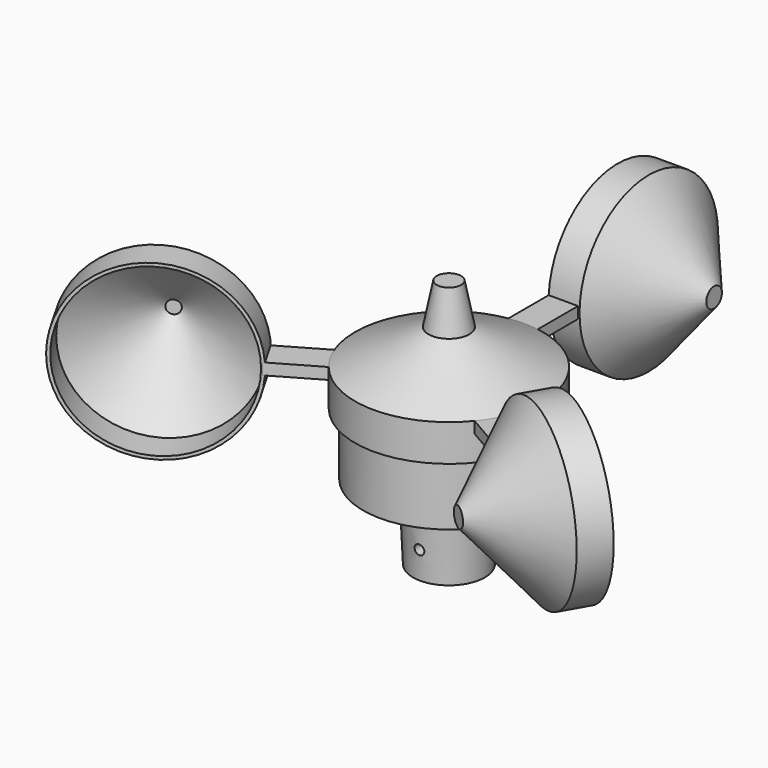
from build123d import *

# Parameters (mm, degrees)
F0_R       = 11
F2_R       = 12
F4_R       = 6.35
F5_R       = 6.35
F7_R       = 26.25
F8_DEPTH   = 19
F9_R       = 28.75
F10_DEPTH  = 9.5
F13_DEPTH  = 1.75
F15_R      = 28.75
F17_DEPTH  = 1.75
F17_FACE_R = 28.75
F16_R      = 6.25
F19_R      = 6.25
F21_R      = 3.75
F23_R      = 26.5
F23_R_2    = 25.5
F24_DEPTH  = 9.5
F27_R      = 26.5
F26_R      = 3
F30_R      = 2
F31_R      = 25.5
F34_COUNT  = 3
F35_R      = 1.5
F36_DEPTH  = 12.5
F37_R      = 6.35
F38_DEPTH  = 9.5


with BuildPart() as f3:
    # F0 (on Top) → F3 section 0
    with BuildSketch(Plane.XY):
        Circle(F0_R)
    # F2 (on offset) → F3 section 1
    with BuildSketch(Plane.XY.offset(23)):
        Circle(F2_R)
    loft()

    # F4 (on face) → F6 section 0
    with BuildSketch(Plane(origin=(0, 0, 0), x_dir=(1, 0, 0), z_dir=(0, 0, -1))):
        Circle(F4_R)
    # F5 (on face) → F6 section 1
    with BuildSketch(Plane.XY.offset(23)):
        Circle(F5_R)
    loft(mode=Mode.SUBTRACT)

    # F7 (on face) → F8 (join)
    with BuildSketch(Plane.XY.offset(23)):
        Circle(F7_R)
    extrude(amount=F8_DEPTH)

    # F9 (on face) → F10 (join)
    with BuildSketch(Plane.XY.offset(42)):
        Circle(F9_R)
    extrude(amount=F10_DEPTH)

    # F12 (on face) → F13 (join, symmetric)
    with BuildSketch(Plane.XY.offset(51.5)):
        Polygon((-4.5, 44.75), (-4.5, 28.3956422713), (-4.5, 22), (4.5, 22), (4.5, 28.3956422713), (4.5, 44.75), (0, 44.75), align=None)
        Polygon((-21.3025588833, -7.102885683), (-26.8413475637, -10.3007068186), (-40.6977540243, -18.3007068186), (-36.1977540243, -26.0949354527), (-22.3413475637, -18.0949354527), (-16.8025588833, -14.897114317), align=None)
        Polygon((16.8025588833, -14.897114317), (22.3413475637, -18.0949354527), (36.1977540243, -26.0949354527), (40.6977540243, -18.3007068186), (26.8413475637, -10.3007068186), (21.3025588833, -7.102885683), align=None)
    extrude(amount=F13_DEPTH, both=True)



with BuildPart() as f17:
    # F15 (on face) → F17 (new body)
    with BuildSketch(Plane.XY.offset(51.5)):
        Circle(F15_R)
    extrude(amount=F17_DEPTH)


with BuildPart() as f18:
    # F17_face (on face) → F18 section 0
    with BuildSketch(Plane.XY.offset(53.25)):
        Circle(F17_FACE_R)
    # F16 (on offset) → F18 section 1
    with BuildSketch(Plane.XY.offset(64)):
        Circle(F16_R)
    loft()


with BuildPart() as f3_1:
    add(f3.part)

    add(f17.part)  # F22 merges F17

    add(f18.part)  # F22 merges F18
    # F19 (on face) → F22 section 0
    with BuildSketch(Plane.XY.offset(64)):
        Circle(F19_R)
    # F21 (on offset) → F22 section 1
    with BuildSketch(Plane.XY.offset(76.5)):
        Circle(F21_R)
    loft()



with BuildPart() as f24:
    # F23 (on face) → F24 (new body)
    with BuildSketch(Plane(origin=(-4.5, 0, 0), x_dir=(0, -1, 0), z_dir=(-1, 0, 0))):
        with Locations((-70.25, 51.5)):
            Circle(F23_R)
        with Locations((-70.25, 51.5)):
            Circle(F23_R_2, mode=Mode.SUBTRACT)
    extrude(amount=-F24_DEPTH)


with BuildPart() as f3_2:
    add(f3_1.part)

    add(f24.part)  # F28 merges F24
    # F27 (on face) → F28 section 0
    with BuildSketch(Plane.YZ.offset(5)):
        with Locations((70.25, 51.5)):
            Circle(F27_R)
    # F26 (on offset) → F28 section 1
    with BuildSketch(Plane.YZ.offset(25)):
        with Locations((70.25, 51.5)):
            Circle(F26_R)
    loft()

    # F30 (on offset) → F32 section 0
    with BuildSketch(Plane.YZ.offset(24)):
        with Locations((70.25, 51.5)):
            Circle(F30_R)
    # F31 (on face) → F32 section 1
    with BuildSketch(Plane(origin=(5, 0, 0), x_dir=(0, -1, 0), z_dir=(-1, 0, 0))):
        with Locations((-70.25, 51.5)):
            Circle(F31_R)
    loft(mode=Mode.SUBTRACT)


with BuildPart() as f34_1:
    # F34: instance of F3
    add(f3_2.part.rotate(Axis((0, 0, 40.5513271689), (0, 0, 1)), 1 * 360 / F34_COUNT))


with BuildPart() as f34_2:
    # F34: instance of F3
    add(f3_2.part.rotate(Axis((0, 0, 40.5513271689), (0, 0, 1)), 2 * 360 / F34_COUNT))


with BuildPart() as f36_tool:
    # F35 (on Front) → F36 (new body, symmetric)
    with BuildSketch(Plane.XZ):
        with Locations((0, 8.5)):
            Circle(F35_R)
    extrude(amount=F36_DEPTH, both=True)


with BuildPart() as f3_3:
    add(f3_2.part)

    # F36: cut by f36_tool
    add(f36_tool.part, mode=Mode.SUBTRACT)



with BuildPart() as f34_1_1:
    add(f34_1.part)

    # F36: cut by f36_tool
    add(f36_tool.part, mode=Mode.SUBTRACT)


with BuildPart() as f34_2_1:
    add(f34_2.part)

    # F36: cut by f36_tool
    add(f36_tool.part, mode=Mode.SUBTRACT)


with BuildPart() as f3_4:
    add(f3_3.part)

    add(f34_1_1.part)  # F38 merges F34_1

    add(f34_2_1.part)  # F38 merges F34_2
    # F37 (on face) → F38 (join)
    with BuildSketch(Plane(origin=(0, 0, 23), x_dir=(1, 0, 0), z_dir=(0, 0, -1))):
        Circle(F37_R)
    extrude(amount=F38_DEPTH)


solid = f3_4.part
